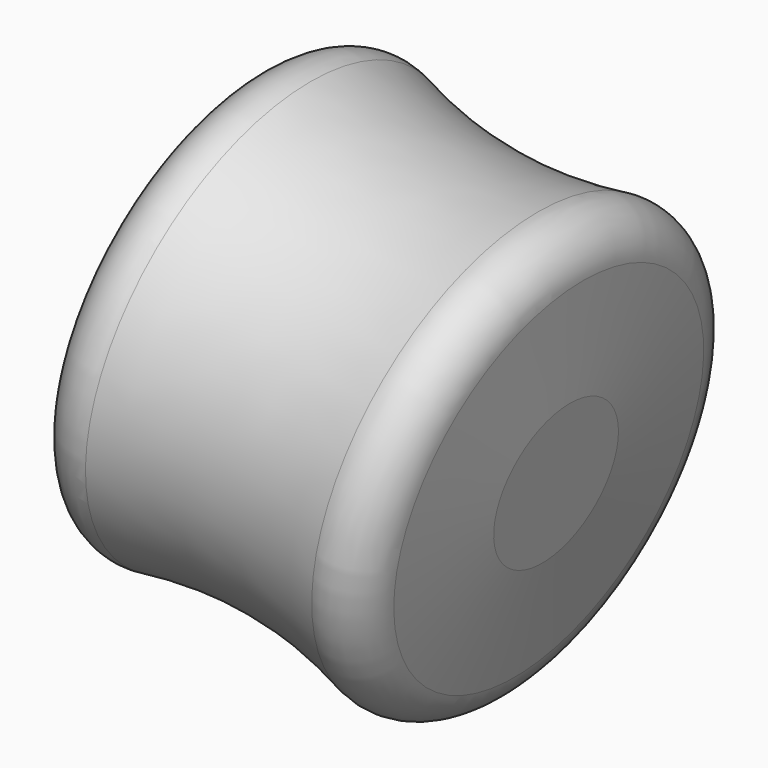
from build123d import *


with BuildPart() as f1:
    # F0 (on Front) → F1 (revolve)
    with BuildSketch(Plane.XZ):
        with BuildLine():
            ThreePointArc((-43.1091779093, -9.5547758593), (-52.0705780398, -9.2030680727), (-60.5916763105, -6.4064138345))
            ThreePointArc((-60.5916763105, -6.4064138345), (-63.4171775016, -6.4207120143), (-65.1124120295, -8.681207826))
            Line((-65.1124120295, -8.681207826), (-66.6337429499, -16.9325878819))
            Line((-66.6337429499, -16.9325878819), (-40.6500098054, -21.7232842734))
            Line((-40.6500098054, -21.7232842734), (-39.6395713434, -13.0827797716))
            ThreePointArc((-39.6395713434, -13.0827797716), (-40.5293607347, -10.487751031), (-43.1091779093, -9.5547758593))
        make_face()
        Polygon((-40.6500098054, -21.7232842734), (-66.6337429499, -16.9325878819), (-67.6951437192, -22.6894031954), (-41.702927998, -27.4816635443), align=None)
    revolve(axis=Axis((-54.6990358586, 0, -25.0855333699), (0.9834247256, 0, -0.1813168746)))


solid = f1.part
